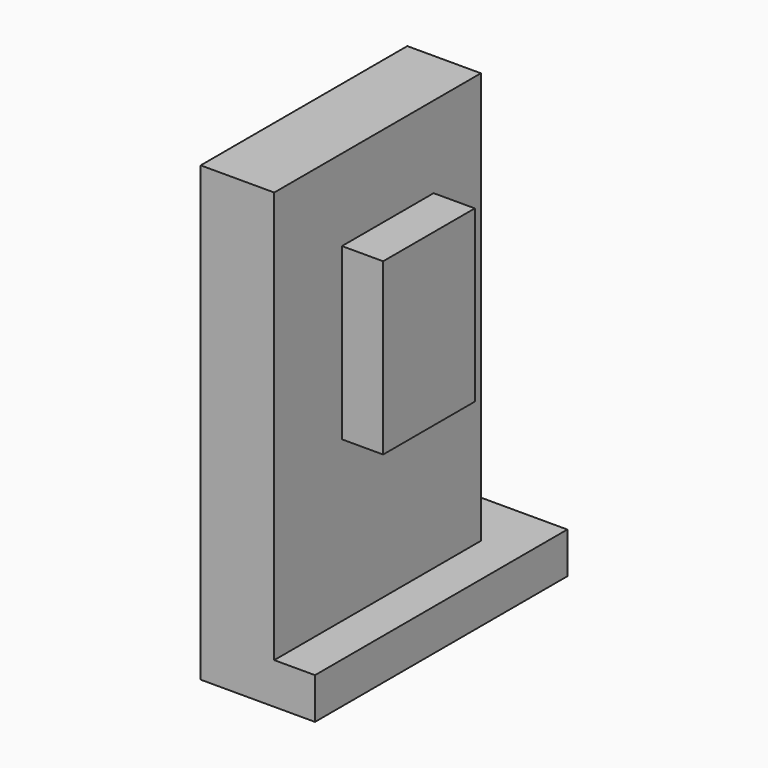
from build123d import *

# Parameters (mm, degrees)
F0_W     = 69.4335103035
F0_H     = 70.5661773682
F1_DEPTH = 25
F2_W     = 44.6875952184
F2_H     = 35.8601175249
F3_DEPTH = 250
F4_DEPTH = 121
F5_W     = 69.5940330625
F5_H     = 103.3312529325
F7_DEPTH = 25


# Not quite as in the source:
# - the program builds the solid bodies; features that only make, move or delete a surface that nothing else refers to are left out


with BuildPart() as f1:
    # F0 (on Top) → F1 (new body)
    with BuildSketch(Plane.XY):
        with Locations((34.7167551517, 35.2830886841)):
            Rectangle(F0_W, F0_H)
    extrude(amount=F1_DEPTH)

    # F2 (on face) → F3 (join)
    with BuildSketch(Plane.XY.offset(25)):
        with Locations((22.3437976092, 17.9300587624)):
            Rectangle(F2_W, F2_H)
    extrude(amount=F3_DEPTH)

    # F4 (add): a face of the model
    f4_faces = [f1.faces().sort_by_distance(p)[0] for p in [
        (24.0077180628, 0, 131.5089430654),
    ]]
    extrude(f4_faces, amount=F4_DEPTH)

    # F5 (on face) → F7 (join)
    with BuildSketch(Plane.YZ.offset(44.6875952184)):
        with Locations((-34.7970165312, 173.8082841039)):
            Rectangle(F5_W, F5_H)
    extrude(amount=F7_DEPTH)


solid = f1.part
